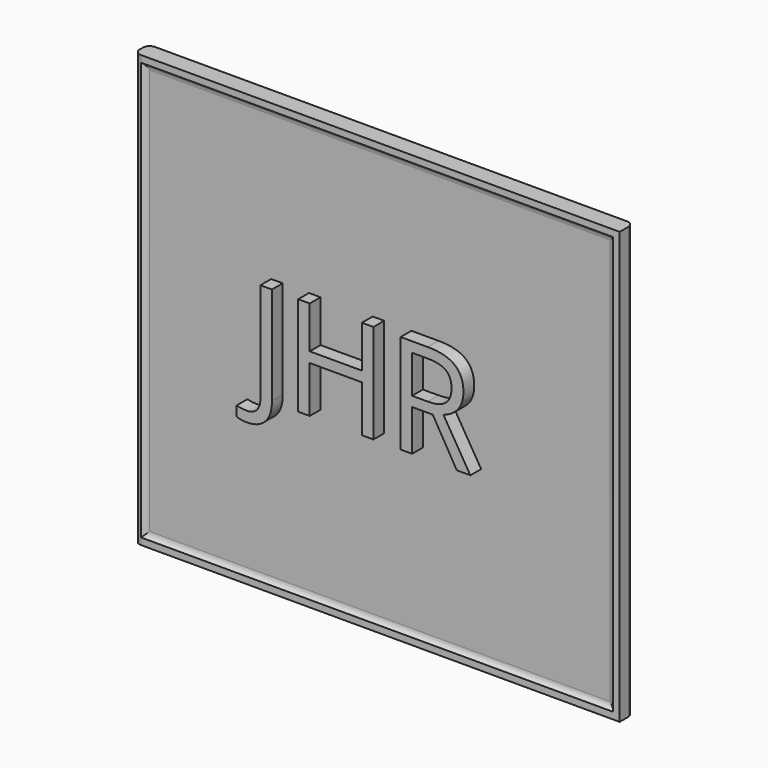
from build123d import *

# Parameters (mm, degrees)
F1_DEPTH      = 320
F2_W          = 350
F2_H          = 310
F3_DEPTH      = 2.5
F4_W          = 84
F4_H          = 65
F5_DEPTH      = 20
F6_SIZE       = 5
F7_T1_DEPTH   = 350
F7_T3_DEPTH   = 310
F7_T9_DEPTH   = 360.8253175473
F7_T13_DEPTH  = 320.8253175473
F7_T20_DEPTH  = 360.8253175473
F7_T24_DEPTH  = 320.8253175473
F7_T31_DEPTH  = 360.8253175473
F7_T35_DEPTH  = 320.8253175473
F7_T42_DEPTH  = 320.8253175473
F7_T46_DEPTH  = 360.8253175473
F8_R          = 12.5
F9_DEPTH      = 20
F10_TEXT_SIZE = 102.9214687751
F11_DEPTH     = 10


# Not quite as in the source:
# - a fillet or chamfer that OpenCascade refuses, or shapes differently, is made with other operations: its cross-section is extruded or revolved along the edge and cut away or added
# - Text() gives the source's letters only with a copy of the font that has no kerning and outlines rounded to 1/6400 em; it was checked with that copy


with BuildPart() as f1:
    # F0 (on Top) → F1 (new body)
    with BuildSketch(Plane.XY):
        with BuildLine():
            Line((175.469207186, 26.9448122531), (-175, 26.9448122531))
            ThreePointArc((-175, 26.9448122531), (-178.5355339059, 25.4803461591), (-180, 21.9448122531))
            Line((-180, 21.9448122531), (-180, 18.9448122531))
            ThreePointArc((-180, 18.9448122531), (-178.5355339059, 15.4092783472), (-175, 13.9448122531))
            Line((-175, 13.9448122531), (180, 13.9448122531))
            Line((180, 13.9448122531), (180, 21.9668764744))
            ThreePointArc((180, 21.9668764744), (178.6977044183, 25.33243468), (175.469207186, 26.9448122531))
        make_face()
    extrude(amount=F1_DEPTH)

    # F2 (on face) → F3 (cut)
    with BuildSketch(Plane.XZ.offset(-13.9448122531)):
        with Locations((0, 160)):
            Rectangle(F2_W, F2_H)
    extrude(amount=-F3_DEPTH, mode=Mode.SUBTRACT)

    # F4 (on face) → F5 (join)
    with BuildSketch(Plane(origin=(0, 26.9448122531, 0), x_dir=(-1, 0, 0), z_dir=(0, 1, 0))):
        with Locations((0, 164.576021559)):
            Rectangle(F4_W, F4_H)
    extrude(amount=F5_DEPTH)

    # F6
    f6_edges = [f1.edges().sort_by_distance(p)[0] for p in [
        (0, 46.944812, 197.076022),
        (42, 46.944812, 164.576022),
        (0, 46.944812, 132.076022),
        (-42, 46.944812, 164.576022),
        (42, 36.944812, 197.076022),
        (42, 36.944812, 132.076022),
        (-42, 36.944812, 132.076022),
        (-42, 36.944812, 197.076022),
    ]]
    chamfer(f6_edges, length=F6_SIZE)

    # F7: fillet of radius 5 on 4 edges, made by hand

    # F7_s2 → F7_t1 (join)
    with BuildSketch(Plane.YZ.offset(-175)):
        with BuildLine():
            ThreePointArc((13.9448122531, 315), (15.774939272, 313.1698729811), (16.4448122531, 310.6698729811))
            Line((16.4448122531, 310.6698729811), (16.5448122531, 310.6698729811))
            Line((16.5448122531, 310.6698729811), (16.5448122531, 315))
            Line((16.5448122531, 315), (16.4448122531, 315.1))
            ThreePointArc((16.4448122531, 315.1), (15.1948122531, 315.1), (13.9948122531, 315.0866025404))
            Line((13.9948122531, 315.0866025404), (13.9448122531, 315))
        make_face()
        with BuildLine():
            ThreePointArc((13.9448122531, 5), (15.774939272, 6.8301270189), (16.4448122531, 9.3301270189))
            Line((16.4448122531, 9.3301270189), (16.5448122531, 9.3301270189))
            Line((16.5448122531, 9.3301270189), (16.5448122531, 5))
            Line((16.5448122531, 5), (16.4448122531, 4.9))
            ThreePointArc((16.4448122531, 4.9), (15.1948122531, 4.9), (13.9948122531, 4.9133974596))
            Line((13.9948122531, 4.9133974596), (13.9448122531, 5))
        make_face()
    extrude(amount=F7_T1_DEPTH)

    # F7_s4 → F7_t3 (join)
    with BuildSketch(Plane.XY.offset(5)):
        with BuildLine():
            ThreePointArc((-175, 13.9448122531), (-173.1698729811, 15.774939272), (-170.6698729811, 16.4448122531))
            Line((-170.6698729811, 16.4448122531), (-170.6698729811, 16.5448122531))
            Line((-170.6698729811, 16.5448122531), (-175, 16.5448122531))
            Line((-175, 16.5448122531), (-175.1, 16.4448122531))
            ThreePointArc((-175.1, 16.4448122531), (-175.1, 15.1948122531), (-175.0866025404, 13.9948122531))
            Line((-175.0866025404, 13.9948122531), (-175, 13.9448122531))
        make_face()
        with BuildLine():
            ThreePointArc((175, 13.9448122531), (173.1698729811, 15.774939272), (170.6698729811, 16.4448122531))
            Line((170.6698729811, 16.4448122531), (170.6698729811, 16.5448122531))
            Line((170.6698729811, 16.5448122531), (175, 16.5448122531))
            Line((175, 16.5448122531), (175.1, 16.4448122531))
            ThreePointArc((175.1, 16.4448122531), (175.1, 15.1948122531), (175.0866025404, 13.9948122531))
            Line((175.0866025404, 13.9948122531), (175, 13.9448122531))
        make_face()
    extrude(amount=F7_T3_DEPTH)


with BuildPart() as f7_tool7:
    # F7_s8 → F7_t9 (new body)
    with BuildSketch(Plane.YZ.offset(185.8253175473)):
        with BuildLine():
            ThreePointArc((13.9448122531, 315), (15.774939272, 313.1698729811), (16.4448122531, 310.6698729811))
            Line((16.4448122531, 310.6698729811), (16.5448122531, 310.6698729811))
            Line((16.5448122531, 310.6698729811), (16.5448122531, 315))
            Line((16.5448122531, 315), (16.4448122531, 315.1))
            ThreePointArc((16.4448122531, 315.1), (15.1948122531, 315.1), (13.9948122531, 315.0866025404))
            Line((13.9948122531, 315.0866025404), (13.9448122531, 315))
        make_face()
    extrude(amount=-F7_T9_DEPTH)

    split(bisect_by=Plane.YZ.offset(175), keep=Keep.TOP)


with BuildPart() as f7_tool11:
    # F7_s12 → F7_t13 (new body)
    with BuildSketch(Plane.XY.offset(5)):
        with BuildLine():
            ThreePointArc((175, 13.9448122531), (173.1698729811, 15.774939272), (170.6698729811, 16.4448122531))
            Line((170.6698729811, 16.4448122531), (170.6698729811, 16.5448122531))
            Line((170.6698729811, 16.5448122531), (175, 16.5448122531))
            Line((175, 16.5448122531), (175.1, 16.4448122531))
            ThreePointArc((175.1, 16.4448122531), (175.1, 15.1948122531), (175.0866025404, 13.9948122531))
            Line((175.0866025404, 13.9948122531), (175, 13.9448122531))
        make_face()
    extrude(amount=F7_T13_DEPTH)

    split(bisect_by=Plane.XY.offset(315), keep=Keep.TOP)


with BuildPart() as f7_tool7_1:
    add(f7_tool7.part)

    # F7_t15: intersect F7_tool11
    add(f7_tool11.part, mode=Mode.INTERSECT)


with BuildPart() as f1_1:
    add(f1.part)

    # F7_t5: union F7_tool7
    add(f7_tool7_1.part)


with BuildPart() as f7_tool18:
    # F7_s19 → F7_t20 (new body)
    with BuildSketch(Plane.YZ.offset(175)):
        with BuildLine():
            ThreePointArc((13.9448122531, 315), (15.774939272, 313.1698729811), (16.4448122531, 310.6698729811))
            Line((16.4448122531, 310.6698729811), (16.5448122531, 310.6698729811))
            Line((16.5448122531, 310.6698729811), (16.5448122531, 315))
            Line((16.5448122531, 315), (16.4448122531, 315.1))
            ThreePointArc((16.4448122531, 315.1), (15.1948122531, 315.1), (13.9948122531, 315.0866025404))
            Line((13.9948122531, 315.0866025404), (13.9448122531, 315))
        make_face()
    extrude(amount=-F7_T20_DEPTH)

    split(bisect_by=Plane.YZ.offset(-175), keep=Keep.BOTTOM)


with BuildPart() as f7_tool22:
    # F7_s23 → F7_t24 (new body)
    with BuildSketch(Plane.XY.offset(325.8253175473)):
        with BuildLine():
            ThreePointArc((-175, 13.9448122531), (-173.1698729811, 15.774939272), (-170.6698729811, 16.4448122531))
            Line((-170.6698729811, 16.4448122531), (-170.6698729811, 16.5448122531))
            Line((-170.6698729811, 16.5448122531), (-175, 16.5448122531))
            Line((-175, 16.5448122531), (-175.1, 16.4448122531))
            ThreePointArc((-175.1, 16.4448122531), (-175.1, 15.1948122531), (-175.0866025404, 13.9948122531))
            Line((-175.0866025404, 13.9948122531), (-175, 13.9448122531))
        make_face()
    extrude(amount=-F7_T24_DEPTH)

    split(bisect_by=Plane.XY.offset(315), keep=Keep.TOP)


with BuildPart() as f7_tool18_1:
    add(f7_tool18.part)

    # F7_t26: intersect F7_tool22
    add(f7_tool22.part, mode=Mode.INTERSECT)


with BuildPart() as f1_2:
    add(f1_1.part)

    # F7_t16: union F7_tool18
    add(f7_tool18_1.part)


with BuildPart() as f7_tool29:
    # F7_s30 → F7_t31 (new body)
    with BuildSketch(Plane.YZ.offset(-185.8253175473)):
        with BuildLine():
            ThreePointArc((13.9448122531, 5), (15.774939272, 6.8301270189), (16.4448122531, 9.3301270189))
            Line((16.4448122531, 9.3301270189), (16.5448122531, 9.3301270189))
            Line((16.5448122531, 9.3301270189), (16.5448122531, 5))
            Line((16.5448122531, 5), (16.4448122531, 4.9))
            ThreePointArc((16.4448122531, 4.9), (15.1948122531, 4.9), (13.9948122531, 4.9133974596))
            Line((13.9948122531, 4.9133974596), (13.9448122531, 5))
        make_face()
    extrude(amount=F7_T31_DEPTH)

    split(bisect_by=Plane.YZ.offset(-175), keep=Keep.BOTTOM)


with BuildPart() as f7_tool33:
    # F7_s34 → F7_t35 (new body)
    with BuildSketch(Plane.XY.offset(315)):
        with BuildLine():
            ThreePointArc((-175, 13.9448122531), (-173.1698729811, 15.774939272), (-170.6698729811, 16.4448122531))
            Line((-170.6698729811, 16.4448122531), (-170.6698729811, 16.5448122531))
            Line((-170.6698729811, 16.5448122531), (-175, 16.5448122531))
            Line((-175, 16.5448122531), (-175.1, 16.4448122531))
            ThreePointArc((-175.1, 16.4448122531), (-175.1, 15.1948122531), (-175.0866025404, 13.9948122531))
            Line((-175.0866025404, 13.9948122531), (-175, 13.9448122531))
        make_face()
    extrude(amount=-F7_T35_DEPTH)

    split(bisect_by=Plane.XY.offset(5), keep=Keep.BOTTOM)


with BuildPart() as f7_tool29_1:
    add(f7_tool29.part)

    # F7_t37: intersect F7_tool33
    add(f7_tool33.part, mode=Mode.INTERSECT)


with BuildPart() as f1_3:
    add(f1_2.part)

    # F7_t27: union F7_tool29
    add(f7_tool29_1.part)


with BuildPart() as f7_tool40:
    # F7_s41 → F7_t42 (new body)
    with BuildSketch(Plane.XY.offset(-5.8253175473)):
        with BuildLine():
            ThreePointArc((175, 13.9448122531), (173.1698729811, 15.774939272), (170.6698729811, 16.4448122531))
            Line((170.6698729811, 16.4448122531), (170.6698729811, 16.5448122531))
            Line((170.6698729811, 16.5448122531), (175, 16.5448122531))
            Line((175, 16.5448122531), (175.1, 16.4448122531))
            ThreePointArc((175.1, 16.4448122531), (175.1, 15.1948122531), (175.0866025404, 13.9948122531))
            Line((175.0866025404, 13.9948122531), (175, 13.9448122531))
        make_face()
    extrude(amount=F7_T42_DEPTH)

    split(bisect_by=Plane.XY.offset(5), keep=Keep.BOTTOM)


with BuildPart() as f7_tool44:
    # F7_s45 → F7_t46 (new body)
    with BuildSketch(Plane.YZ.offset(-175)):
        with BuildLine():
            ThreePointArc((13.9448122531, 5), (15.774939272, 6.8301270189), (16.4448122531, 9.3301270189))
            Line((16.4448122531, 9.3301270189), (16.5448122531, 9.3301270189))
            Line((16.5448122531, 9.3301270189), (16.5448122531, 5))
            Line((16.5448122531, 5), (16.4448122531, 4.9))
            ThreePointArc((16.4448122531, 4.9), (15.1948122531, 4.9), (13.9948122531, 4.9133974596))
            Line((13.9948122531, 4.9133974596), (13.9448122531, 5))
        make_face()
    extrude(amount=F7_T46_DEPTH)

    split(bisect_by=Plane.YZ.offset(175), keep=Keep.TOP)


with BuildPart() as f7_tool40_1:
    add(f7_tool40.part)

    # F7_t48: intersect F7_tool44
    add(f7_tool44.part, mode=Mode.INTERSECT)


with BuildPart() as f1_4:
    add(f1_3.part)

    # F7_t38: union F7_tool40
    add(f7_tool40_1.part)

    # F8 (on face) → F9 (cut)
    with BuildSketch(Plane(origin=(0, 46.9448122531, 0), x_dir=(-1, 0, 0), z_dir=(0, 1, 0))):
        with Locations((0, 164.576021559)):
            Circle(F8_R)
    extrude(amount=-F9_DEPTH, mode=Mode.SUBTRACT)

    # F10 (on face) → F11 (join)
    with BuildSketch(Plane.XZ.offset(-16.4448122531)):
        with Locations((-90, 130.0151537951)):
            Text('JHR', F10_TEXT_SIZE, font='Open Sans', text_align=(TextAlign.LEFT, TextAlign.BOTTOM))
    extrude(amount=F11_DEPTH)


solid = f1_4.part
